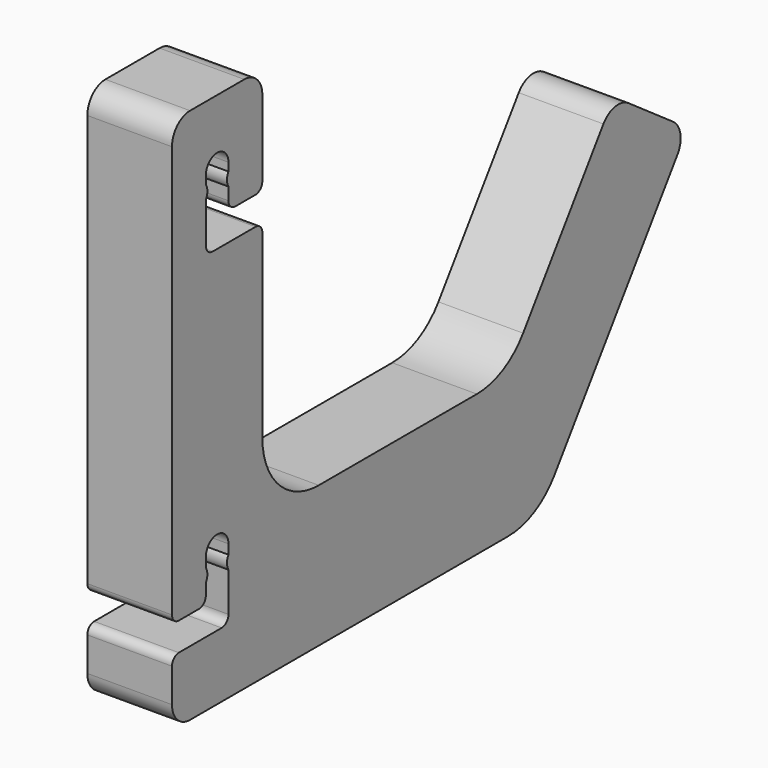
from build123d import *

# Parameters (mm, degrees)
F1_DEPTH = 3.81
F2_R     = 2.032
F4_DEPTH = 7.621
F5_R     = 0.762
F7_DEPTH = 7.62


# Not quite as in the source:
# - a feature names something its author has since deleted; it is built from what else it names


with BuildPart() as f1:
    # F0 (on Right) → F1 (new body, symmetric)
    with BuildSketch(Plane.YZ):
        with BuildLine():
            Line((0, 43.18), (0, 0))
            Line((0, 0), (0, -5.08))
            Line((0, -5.08), (37.8004340866, -5.08))
            ThreePointArc((37.8004340866, -5.08), (40.7325377806, -4.3625187907), (43.0020495678, -2.3722103708))
            Line((43.0020495678, -2.3722103708), (58.0123892895, 19.0647763833))
            Line((58.0123892895, 19.0647763833), (49.6898045196, 24.8923129766))
            Line((49.6898045196, 24.8923129766), (39.4916154812, 10.3277896292))
            ThreePointArc((39.4916154812, 10.3277896292), (37.222103694, 8.3374812093), (34.29, 7.62))
            Line((34.29, 7.62), (16.51, 7.62))
            ThreePointArc((16.51, 7.62), (12.0198719395, 9.4798719395), (10.16, 13.97))
            Line((10.16, 13.97), (10.16, 43.18))
            Line((10.16, 43.18), (0, 43.18))
        make_face()
    extrude(amount=F1_DEPTH, both=True)

    # F2
    f2_edges = [f1.edges().sort_by_distance(p)[0] for p in [
        (0, 10.16, 43.18),
        (0, 0, 43.18),
        (0, 49.689805, 24.892313),
        (0, 58.012389, 19.064776),
        (0, 0, -5.08),
    ]]
    fillet(f2_edges, radius=F2_R)

    # F3 (on face) → F4 (cut, through all)
    with BuildSketch(Plane.YZ.offset(3.81)):
        with BuildLine():
            Line((6.35, 33.528), (6.35, 37.338))
            ThreePointArc((6.35, 37.338), (5.08, 38.608), (3.81, 37.338))
            Line((3.81, 37.338), (3.81, 30.988))
            Line((3.81, 30.988), (10.16, 30.988))
            Line((10.16, 30.988), (10.16, 33.528))
            Line((10.16, 33.528), (6.35, 33.528))
        make_face()
        with BuildLine():
            Line((6.35, 0.762), (6.35, 7.112))
            ThreePointArc((6.35, 7.112), (5.08, 8.382), (3.81, 7.112))
            Line((3.81, 7.112), (3.81, 3.302))
            Line((3.81, 3.302), (0, 3.302))
            Line((0, 3.302), (0, 0.762))
            Line((0, 0.762), (6.35, 0.762))
        make_face()
    extrude(amount=-F4_DEPTH, mode=Mode.SUBTRACT)

    # F5
    f5_edges = [f1.edges().sort_by_distance(p)[0] for p in [
        (0, 6.35, 33.528),
        (0, 10.16, 33.528),
        (0, 3.81, 30.988),
        (0, 10.16, 30.988),
        (0, 0, 3.302),
        (0, 6.35, 0.762),
        (0, 0, 0.762),
        (0, 3.81, 3.302),
    ]]
    fillet(f5_edges, radius=F5_R)

    # F6 (on face) → F7 (join, through all)
    with BuildSketch(Plane.YZ.offset(3.81)):
        with BuildLine():
            Line((6.35, 35.4090145557), (6.35, 36.6031861632))
            ThreePointArc((6.35, 36.6031861632), (6.1816473942, 36.0061003594), (6.35, 35.4090145557))
        make_face()
        with BuildLine():
            Line((3.81, 36.6031861632), (3.81, 35.4090145557))
            ThreePointArc((3.81, 35.4090145557), (3.9783526058, 36.0061003594), (3.81, 36.6031861632))
        make_face()
        with BuildLine():
            Line((3.81, 6.2505925306), (3.81, 5.0564209231))
            ThreePointArc((3.81, 5.0564209231), (3.9783526058, 5.6535067269), (3.81, 6.2505925306))
        make_face()
        with BuildLine():
            ThreePointArc((6.35, 6.2505925306), (6.1816473942, 5.6535067269), (6.35, 5.0564209231))
            Line((6.35, 5.0564209231), (6.35, 6.2505925306))
        make_face()
    extrude(amount=-F7_DEPTH)


solid = f1.part
